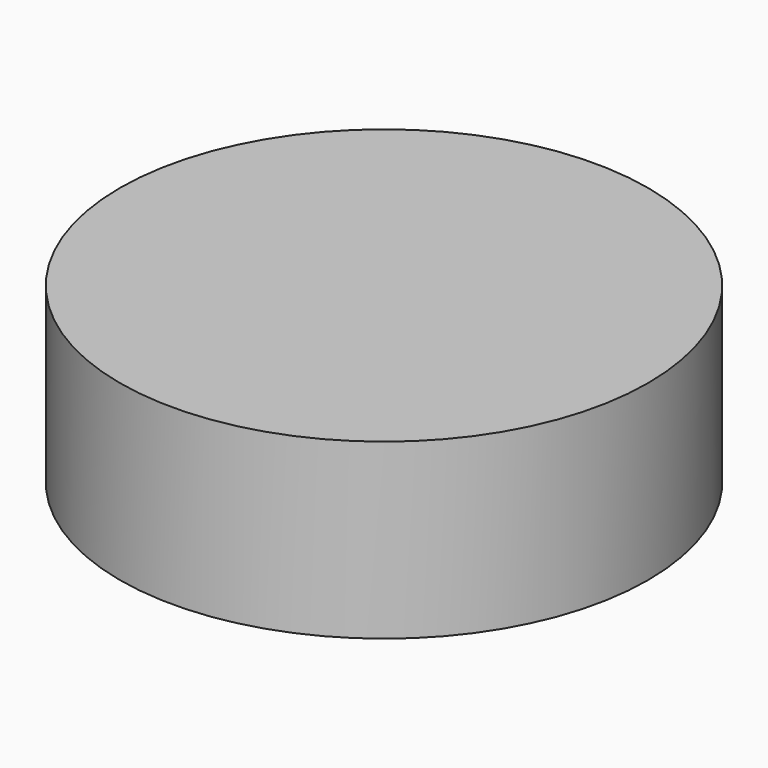
from build123d import *

# Parameters (mm, degrees)
F1_R     = 27.0733874143
F4_DEPTH = 17.78


# Not quite as in the source:
# - the program builds the solid bodies; features that only make, move or delete a surface that nothing else refers to are left out


with BuildPart() as f4:
    # F1 (on face) → F4 (new body)
    with BuildSketch(Plane.XY):
        Circle(F1_R)
    extrude(amount=-F4_DEPTH)


solid = f4.part
